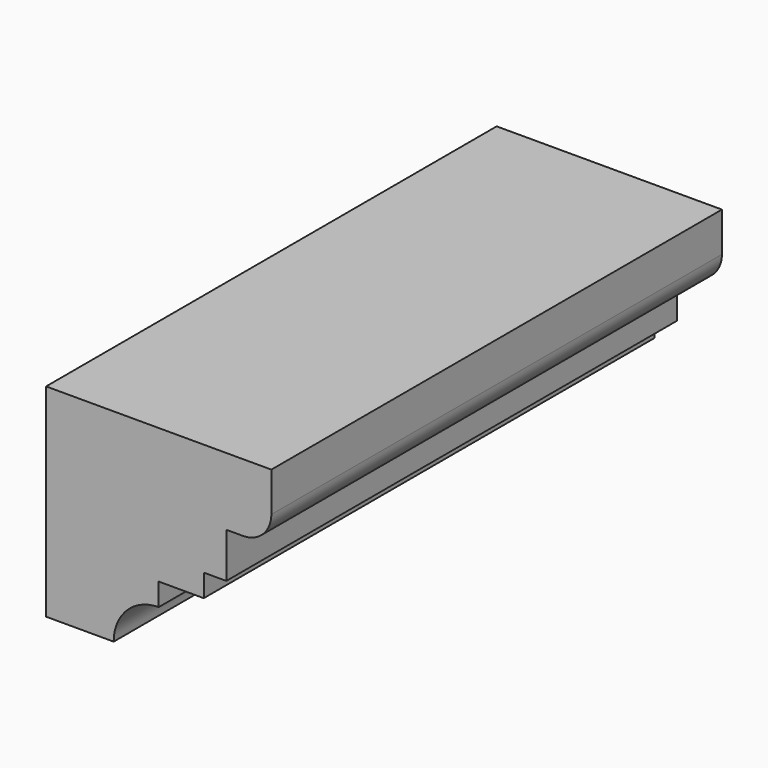
from build123d import *

# Parameters (mm, degrees)
F1_DEPTH = 25


# Not quite as in the source:
# - a feature names something its author has since deleted; it is built from what else it names


with BuildPart() as f1:
    # F0 (on Front) → F1 (new body, symmetric)
    with BuildSketch(Plane.XZ):
        with BuildLine():
            Line((36, 6), (36, 0))
            Line((36, 0), (52, 0))
            Line((52, 0), (53.5, 0))
            ThreePointArc((53.5, 0), (55.267766953, 0.732233047), (56, 2.5))
            Line((56, 2.5), (56, 6))
            Line((56, 6), (36, 6))
        make_face()
        Polygon((52, 0), (36, 0), (36, -4), (50, -4), (52, -4), align=None)
        Polygon((50, -4), (36, -4), (36, -6), (46, -6), (50, -6), align=None)
        with BuildLine():
            Line((46, -6), (36, -6))
            Line((36, -6), (36, -12))
            Line((36, -12), (42, -12))
            ThreePointArc((42, -12), (43.1715728753, -9.1715728753), (46, -8))
            Line((46, -8), (46, -6))
        make_face()
    extrude(amount=F1_DEPTH, both=True)


solid = f1.part
